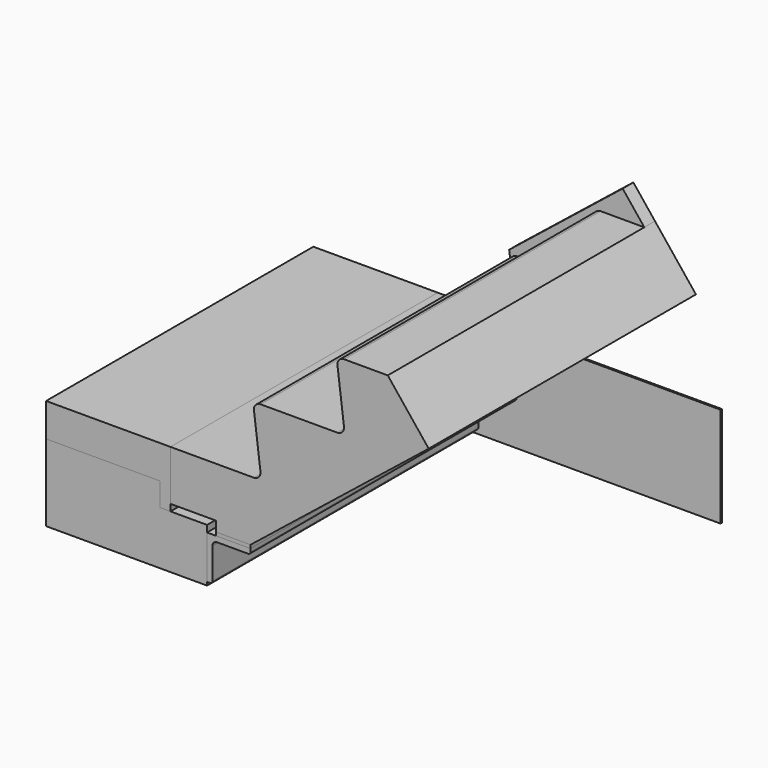
from build123d import *

# Parameters (mm, degrees)
F1_DEPTH = 1000
F2_DEPTH = 1000
F3_DEPTH = 1000
F4_DEPTH = 40
F5_DEPTH = 1000
F0_W     = 103.16486
F0_H     = 10
F6_DEPTH = 1000
F7_DEPTH = 5


# Not quite as in the source:
# - ends of sketch curves that miss each other by under 0.0002 mm in the source are joined


with BuildPart() as f1:
    # F0 (on Front) → F1 (new body)
    with BuildSketch(Plane.XZ):
        Polygon((-148.679091, -189.326917), (-258.2703, -189.326917), (-290.006736, -189.326917), (-290.006736, -119.326917), (-630.630191, -119.326917), (-630.630191, -299.326917), (-148.679091, -299.326917), (-148.679091, -209.326917), align=None)
        Polygon((-148.679091, -299.326917), (-630.630191, -299.326917), (-630.630191, -349.326917), (-148.679091, -349.326917), (-148.679091, -339.326917), align=None)
    extrude(amount=F1_DEPTH)


with BuildPart() as f2:
    # F0 (on Front) → F2 (new body)
    with BuildSketch(Plane.XZ):
        Polygon((-258.2703, -169.326917), (-258.2703, -19.326917), (-630.630191, -19.326917), (-630.630191, -119.326917), (-290.006736, -119.326917), (-290.006736, -189.326917), (-258.2703, -189.326917), align=None)
    extrude(amount=F2_DEPTH)


with BuildPart() as f3:
    # F0 (on Front) → F3 (new body)
    with BuildSketch(Plane.XZ):
        with BuildLine():
            Line((-8.736031, -19.326917), (-258.2703, -19.326917))
            Line((-258.2703, -19.326917), (-258.2703, -169.326917))
            Line((-258.2703, -169.326917), (-148.679091, -169.326917))
            Line((-148.679091, -169.326917), (-121.843951, -169.326917))
            Line((-121.843951, -169.326917), (-121.843951, -199.326917))
            Line((-121.843951, -199.326917), (-18.679091, -199.326917))
            Line((-18.679091, -199.326917), (168.8209090686, -49.3269170857))
            Line((168.8209090686, -49.3269170857), (514.767742, 227.430549))
            Line((514.767742, 227.430549), (392.2610169622, 380.6730829698))
            Line((392.2610169622, 380.6730829698), (261.575257, 380.673083))
            ThreePointArc((261.575257, 380.673083), (246.5816933606, 373.9091341252), (241.7296995119, 358.192387939))
            Line((241.7296995119, 358.192387939), (261.109526, 203.153777))
            ThreePointArc((261.109526, 203.153777), (256.2575323111, 187.4370315028), (241.263969, 180.673083))
            Line((241.263969, 180.673083), (11.575257, 180.673083))
            ThreePointArc((11.575257, 180.673083), (-3.4183066394, 173.9091341252), (-8.2703004881, 158.192387939))
            Line((-8.2703004881, 158.192387939), (11.109526, 3.153777))
            ThreePointArc((11.109526, 3.153777), (6.2575323111, -12.5629684972), (-8.736031, -19.326917))
        make_face()
    extrude(amount=F3_DEPTH)


with BuildPart() as f4:
    # F0 (on Front) → F4 (new body)
    with BuildSketch(Plane.XZ):
        with BuildLine():
            Line((-12.247023, 190.006168), (-8.2703004714, 158.1923879411))
            ThreePointArc((-8.2703004714, 158.1923879411), (-3.4183066394, 173.9091341252), (11.575257, 180.673083))
            Line((11.575257, 180.673083), (241.263969, 180.673083))
            ThreePointArc((241.263969, 180.673083), (256.2575323111, 187.4370315028), (261.1095266112, 203.1537770764))
            Line((261.1095266112, 203.1537770764), (241.7297, 358.192388))
            ThreePointArc((241.7297, 358.192388), (246.5816933606, 373.9091341252), (261.575257, 380.673083))
            Line((261.575257, 380.673083), (392.261017, 380.673083))
            Line((392.261017, 380.673083), (327.4406389587, 461.756296967))
            Line((327.4406389587, 461.756296967), (-12.247023, 190.006168))
        make_face()
    extrude(amount=F4_DEPTH)


with BuildPart() as f5:
    # F0 (on Front) → F5 (new body)
    with BuildSketch(Plane.XZ):
        with BuildLine():
            Line((-121.843951, -209.326917), (-148.679091, -209.326917))
            Line((-148.679091, -209.326917), (-148.679091, -299.326917))
            Line((-148.679091, -299.326917), (-148.679091, -339.326917))
            Line((-148.679091, -339.326917), (-139.679091, -339.326917))
            ThreePointArc((-139.679091, -339.326917), (-134.7293435317, -337.2766644683), (-132.679091, -332.326917))
            Line((-132.679091, -332.326917), (-132.679091, -239.326917))
            ThreePointArc((-132.679091, -239.326917), (-128.5785859366, -229.4274220634), (-118.679091, -225.326917))
            Line((-118.679091, -225.326917), (-25.679091, -225.326917))
            ThreePointArc((-25.679091, -225.326917), (-20.7293435317, -223.2766644683), (-18.679091, -218.326917))
            Line((-18.679091, -218.326917), (-18.679091, -209.326917))
            Line((-18.679091, -209.326917), (-121.843951, -209.326917))
        make_face()
    extrude(amount=F5_DEPTH)


with BuildPart() as f6:
    # F0 (on Front) → F6 (new body)
    with BuildSketch(Plane.XZ):
        with Locations((-70.261521, -204.326917)):
            Rectangle(F0_W, F0_H)
    extrude(amount=F6_DEPTH)


with BuildPart() as f7:
    # F0 (on Front) → F7 (new body)
    with BuildSketch(Plane.XZ):
        with BuildLine():
            Line((168.8209090686, -49.3269170857), (-18.679091, -199.326917))
            Line((-18.679091, -199.326917), (-18.679091, -209.326917))
            Line((-18.679091, -209.326917), (-18.679091, -218.326917))
            ThreePointArc((-18.679091, -218.326917), (-20.7293435317, -223.2766644683), (-25.679091, -225.326917))
            Line((-25.679091, -225.326917), (-118.679091, -225.326917))
            ThreePointArc((-118.679091, -225.326917), (-128.5785859366, -229.4274220634), (-132.679091, -239.326917))
            Line((-132.679091, -239.326917), (-132.679091, -332.326917))
            ThreePointArc((-132.679091, -332.326917), (-134.7293435317, -337.2766644683), (-139.679091, -339.326917))
            Line((-139.679091, -339.326917), (-148.679091, -339.326917))
            Line((-148.679091, -339.326917), (-148.679091, -349.326917))
            Line((-148.679091, -349.326917), (592.581942, -349.326917))
            Line((592.581942, -349.326917), (592.581942, -49.326917))
            Line((592.581942, -49.326917), (168.8209090686, -49.3269170857))
        make_face()
    extrude(amount=F7_DEPTH)


solid = Compound([f1.part, f2.part, f3.part, f4.part, f5.part, f6.part, f7.part])
